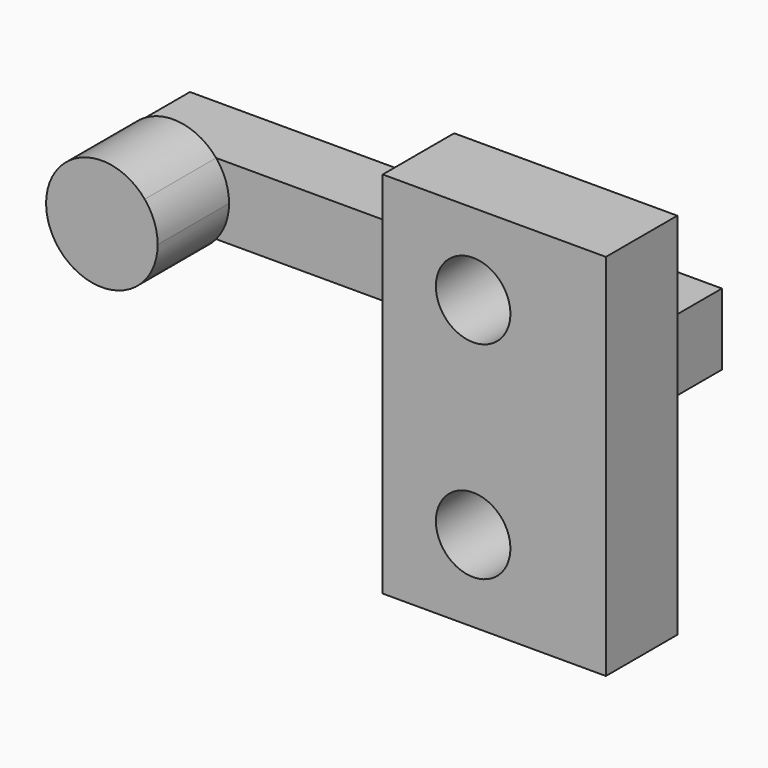
from build123d import *

# Parameters (mm, degrees)
F0_W      = 7.3153038846
F0_H      = 6.1001601681
F1_DEPTH  = 7.62
F2_DEPTH  = 6.35
F3_DEPTH  = 25.4
F4_DEPTH  = 6.35
F5_DEPTH  = 6.35
F6_DEPTH  = 7.62
F7_DEPTH  = 12.7
F8_DEPTH  = 12.7
F9_DEPTH  = 12.7
F10_DEPTH = 6.35
F11_R     = 3.1800137538
F12_DEPTH = 25.4


with BuildPart() as f1:
    # F0 (on Front) → F1 (new body)
    with BuildSketch(Plane.XZ):
        with BuildLine():
            ThreePointArc((3.6576519423, -3.0500800841), (4.4777769945, -1.622010924), (4.7625, 0))
            ThreePointArc((4.7625, 0), (4.4777769945, 1.622010924), (3.6576519423, 3.0500800841))
            Line((3.6576519423, 3.0500800841), (3.6576519423, -3.0500800841))
        make_face()
        with BuildLine():
            Line((-3.6576519423, 3.0500800841), (3.6576519423, 3.0500800841))
            ThreePointArc((3.6576519423, 3.0500800841), (0, 4.7625), (-3.6576519423, 3.0500800841))
        make_face()
        Rectangle(F0_W, F0_H)
        with BuildLine():
            ThreePointArc((-3.6576519423, -3.0500800841), (0, -4.7625), (3.6576519423, -3.0500800841))
            Line((3.6576519423, -3.0500800841), (-3.6576519423, -3.0500800841))
        make_face()
        with BuildLine():
            Line((-3.6576519423, -3.0500800841), (-3.6576519423, 3.0500800841))
            ThreePointArc((-3.6576519423, 3.0500800841), (-4.7625, 0), (-3.6576519423, -3.0500800841))
        make_face()
    extrude(amount=F1_DEPTH)

    # F0 (on Front) → F2 (join)
    with BuildSketch(Plane.XZ):
        Rectangle(F0_W, F0_H)
    extrude(amount=-F2_DEPTH)

    # F3 (add): a face of the model
    f3_faces = [f1.faces().sort_by_distance(p)[0] for p in [
        (3.6576519423, 3.175, 0),
    ]]
    extrude(f3_faces, amount=F3_DEPTH)


with BuildPart() as f4:
    # F4 (new): a face of the model
    f4_faces = [f1.part.faces().sort_by_distance(p)[0] for p in [
        (29.0576519423, 3.175, 0),
    ]]
    extrude(f4_faces, amount=F4_DEPTH)

    # F5 (add): a face of the model
    f5_faces = [f4.faces().sort_by_distance(p)[0] for p in [
        (32.2326519423, 0, 0),
    ]]
    extrude(f5_faces, amount=F5_DEPTH)


with BuildPart() as f6:
    # F6 (new): a face of the model
    f6_faces = [f4.part.faces().sort_by_distance(p)[0] for p in [
        (32.2326519423, -6.35, 0),
    ]]
    extrude(f6_faces, amount=F6_DEPTH)

    # F7 (add): a face of the model
    f7_faces = [f6.faces().sort_by_distance(p)[0] for p in [
        (35.4076519423, -10.16, 0),
    ]]
    extrude(f7_faces, amount=F7_DEPTH)

    # F8 (add): a face of the model
    f8_faces = [f6.faces().sort_by_distance(p)[0] for p in [
        (38.5826519423, -10.16, -3.0500800841),
    ]]
    extrude(f8_faces, amount=F8_DEPTH)

    # F9 (add): a face of the model
    f9_faces = [f6.faces().sort_by_distance(p)[0] for p in [
        (38.5826519423, -10.16, 3.0500800841),
    ]]
    extrude(f9_faces, amount=F9_DEPTH)

    # F11 (on face) → F12 (cut)
    with BuildSketch(Plane(origin=(0, -6.35, 0), x_dir=(-1, 0, 0), z_dir=(0, 1, 0))):
        with Locations((-36.7744378746, 8.8227791712)):
            Circle(F11_R)
        with Locations((-36.7744378746, -8.8227791712)):
            Circle(F11_R)
    extrude(amount=-F12_DEPTH, mode=Mode.SUBTRACT)


with BuildPart() as f10:
    # F10 (new): a face of the model
    f10_faces = [f4.part.faces().sort_by_distance(p)[0] for p in [
        (35.4076519423, 0, 0),
    ]]
    extrude(f10_faces, amount=F10_DEPTH)


solid = Compound([f1.part, f4.part, f6.part, f10.part])
